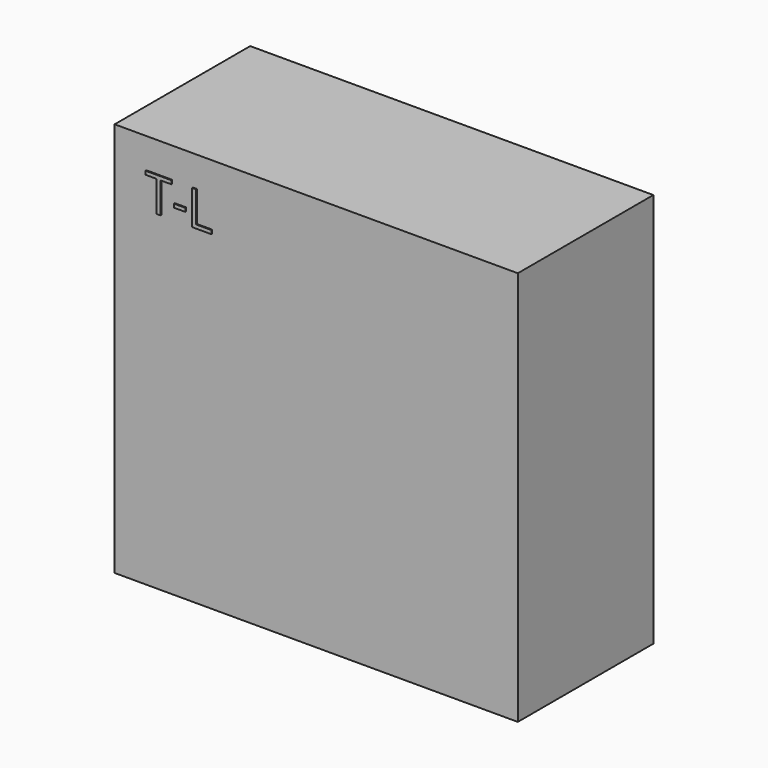
from build123d import *

# Parameters (mm, degrees)
F0_W         = 2425.7
F0_H         = 1019.175
F1_DEPTH     = 2376.4875
F2_TEXT_SIZE = 290.5395295885
F3_DEPTH     = 6.35


# Not quite as in the source:
# - Text() gives the source's letters only with a copy of the font that has no kerning and outlines rounded to 1/6400 em; it was checked with that copy


with BuildPart() as f1:
    # F0 (on Top) → F1 (new body)
    with BuildSketch(Plane.XY):
        with Locations((1212.85, 509.5875)):
            Rectangle(F0_W, F0_H)
    extrude(amount=F1_DEPTH)

    # F2 (on face) → F3 (join)
    with BuildSketch(Plane.XZ):
        with Locations((188.0128085613, 1987.7116680145)):
            Text('T-L', F2_TEXT_SIZE, font='Open Sans', text_align=(TextAlign.LEFT, TextAlign.BOTTOM))
    extrude(amount=F3_DEPTH)


solid = f1.part
